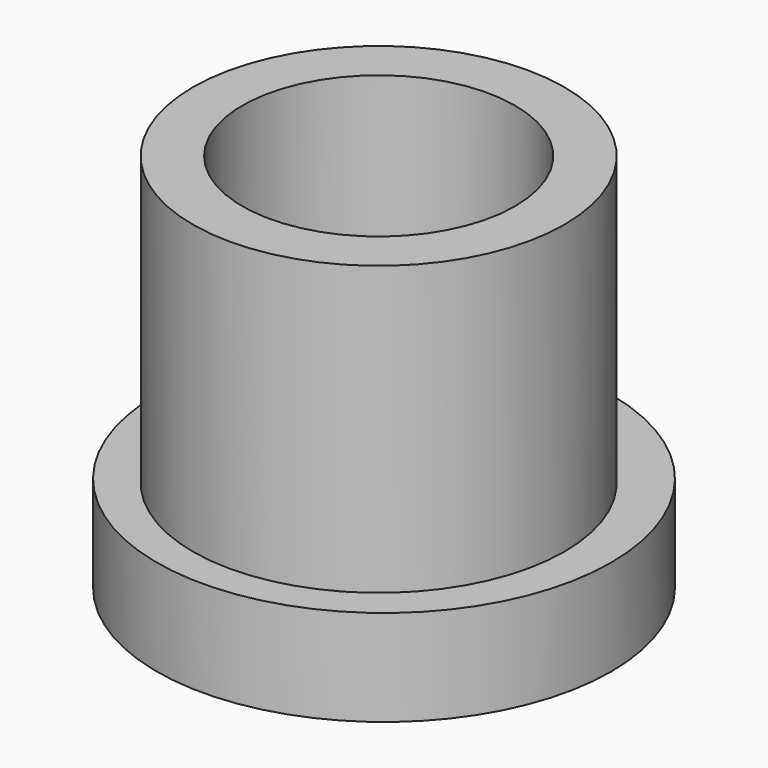
from build123d import *

# Parameters (mm, degrees)
F0_R     = 83.5800069383
F0_R_2   = 61.6002639071
F1_DEPTH = 381
F2_DEPTH = 127
F4_R     = 48.4229343949
F4_R_2   = 35.527059512
F5_DEPTH = 100
F6_R     = 59.1924644961
F7_DEPTH = 25


with BuildPart() as f1:
    # F0 (on Top) → F1 (new body)
    with BuildSketch(Plane.XY):
        with Locations((-408.8018536568, 0)):
            Circle(F0_R)
        with Locations((-408.8018536568, 0)):
            Circle(F0_R_2, mode=Mode.SUBTRACT)
    extrude(amount=F1_DEPTH)

    # F2 (add): a face of the model
    f2_faces = [f1.faces().sort_by_distance(p)[0] for p in [
        (-490.0178610079, 0, 381),
    ]]
    extrude(f2_faces, amount=F2_DEPTH)


with BuildPart() as f5:
    # F4 (on Top) → F5 (new body)
    with BuildSketch(Plane.XY):
        with Locations((-174.1937100887, 12.2994268313)):
            Circle(F4_R)
        with Locations((-174.1937100887, 12.2994268313)):
            Circle(F4_R_2, mode=Mode.SUBTRACT)
    extrude(amount=F5_DEPTH)

    # F6 (on Top) → F7 (join)
    with BuildSketch(Plane.XY):
        with Locations((-174.5279580355, 14.4501468167)):
            Circle(F6_R)
    extrude(amount=F7_DEPTH)


solid = f5.part
